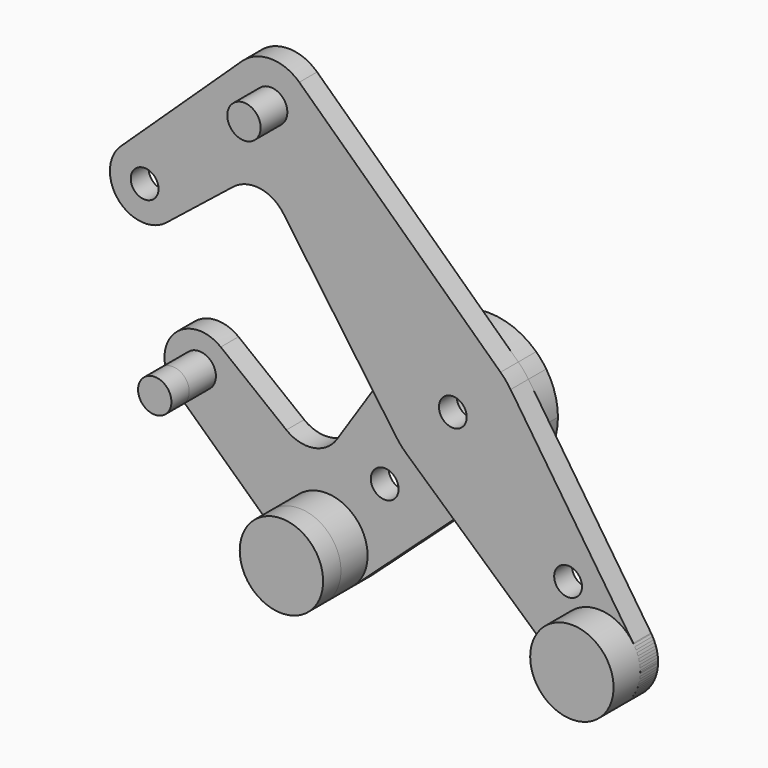
from build123d import *

# Parameters (mm, degrees)
F0_R     = 3.175
F0_R_2   = 3.96875
F2_DEPTH = 5.08
F3_DEPTH = 5.08
F4_R     = 3.81
F6_DEPTH = 12.7
F4_R_2   = 9.525
F5_R     = 3.81
F5_R_2   = 9.525


# Not quite as in the source:
# - a pattern or mirror of a feature is missing from the dataset's text; its kind, count and spacing are read off the source's solid


with BuildPart() as f2:
    # F0 (on Front) → F2 (new body)
    with BuildSketch(Plane.XZ):
        with BuildLine():
            ThreePointArc((-62.4511918078, 23.0063483758), (-67.2442419203, 30.2944442282), (-75.8348368232, 28.7807237291))
            ThreePointArc((-75.8348368232, 28.7807237291), (-76.3849752141, 17.8055319436), (-65.4422370763, 16.798571653))
            ThreePointArc((-65.4422370763, 16.798571653), (-63.237943921, 19.5609585706), (-62.4511918078, 23.0063483758))
        make_face()
        with Locations((-70.3886918078, 23.0063483758)):
            Circle(F0_R, mode=Mode.SUBTRACT)
        with BuildLine():
            ThreePointArc((-13.2524193062, 8.7400805221), (-1.834314477, 15.7686687897), (10.8922900307, 11.5487507067))
            Line((10.8922900307, 11.5487507067), (-35.0711574392, 54.8995176744))
            ThreePointArc((-35.0711574392, 54.8995176744), (-32.8608164346, 51.7436071154), (-32.0815314576, 47.9702672503))
            ThreePointArc((-32.0815314576, 47.9702672503), (-45.3798713227, 39.2245522274), (-48.1419054761, 54.8995176744))
            Line((-48.1419054761, 54.8995176744), (-75.8348368232, 28.7807237291))
            ThreePointArc((-75.8348368232, 28.7807237291), (-67.2442419203, 30.2944442282), (-62.4511918078, 23.0063483758))
            ThreePointArc((-62.4511918078, 23.0063483758), (-63.237943921, 19.5609585706), (-65.4422370763, 16.798571653))
            Line((-65.4422370763, 16.798571653), (-50.1509863937, 28.9828821829))
            ThreePointArc((-50.1509863937, 28.9828821829), (-44.0823996147, 30.6328866939), (-38.7182233604, 27.3502241323))
            Line((-38.7182233604, 27.3502241323), (-19.2147683858, -0.3005169703))
            Line((-19.2147683858, -0.3005169703), (-13.2524193062, 8.7400805221))
        make_face()
        with BuildLine():
            ThreePointArc((-32.0815314576, 47.9702672503), (-32.8608164346, 51.7436071154), (-35.0711574392, 54.8995176744))
            ThreePointArc((-35.0711574392, 54.8995176744), (-41.6065314576, 57.4952672503), (-48.1419054761, 54.8995176744))
            ThreePointArc((-48.1419054761, 54.8995176744), (-45.3798713227, 39.2245522274), (-32.0815314576, 47.9702672503))
        make_face()
        with Locations((-41.6065314576, 47.9702672503)):
            Circle(F0_R, mode=Mode.SUBTRACT)
        with BuildLine():
            ThreePointArc((15.875, 0), (15.1912005478, 4.609018433), (13.1987101208, 8.820979319))
            ThreePointArc((13.1987101208, 8.820979319), (12.1224690662, 10.2499448164), (10.8922900307, 11.5487507067))
            ThreePointArc((10.8922900307, 11.5487507067), (-1.834314477, 15.7686687897), (-13.2524193062, 8.7400805221))
            ThreePointArc((-13.2524193062, 8.7400805221), (-15.8730587934, -0.2482529814), (-12.9726166036, -9.1502373442))
            ThreePointArc((-12.9726166036, -9.1502373442), (-11.8607666217, -10.5516747555), (-10.5983019047, -11.8191210221))
            ThreePointArc((-10.5983019047, -11.8191210221), (0.0485522706, -15.8749257534), (10.6703987497, -11.7540722953))
            ThreePointArc((10.6703987497, -11.7540722953), (14.5156502636, -6.4274040191), (15.875, 0))
        make_face()
        Circle(F0_R_2, mode=Mode.SUBTRACT)
        with BuildLine():
            ThreePointArc((-12.9726166036, -9.1502373442), (-15.8730587934, -0.2482529814), (-13.2524193062, 8.7400805221))
            Line((-13.2524193062, 8.7400805221), (-19.2147683858, -0.3005169703))
            Line((-19.2147683858, -0.3005169703), (-12.9726166036, -9.1502373442))
        make_face()
        with BuildLine():
            Line((-10.5983019047, -11.8191210221), (0.0653932355, -21.3813431455))
            Line((0.0653932355, -21.3813431455), (10.6703987497, -11.7540722953))
            ThreePointArc((10.6703987497, -11.7540722953), (0.0485522706, -15.8749257534), (-10.5983019047, -11.8191210221))
        make_face()
        with BuildLine():
            ThreePointArc((26.9262440233, -45.4676864135), (27.0442454474, -31.1806737127), (41.2044512386, -33.0836262089))
            Line((41.2044512386, -33.0836262089), (13.1987101208, 8.820979319))
            ThreePointArc((13.1987101208, 8.820979319), (15.1912005478, 4.609018433), (15.875, 0))
            ThreePointArc((15.875, 0), (14.5156502636, -6.4274040191), (10.6703987497, -11.7540722953))
            Line((10.6703987497, -11.7540722953), (0.0653932355, -21.3813431455))
            Line((0.0653932355, -21.3813431455), (26.9262440233, -45.4676864135))
        make_face()
        with Locations((26.3222689506, -25.5025770961)):
            Circle(F0_R, mode=Mode.SUBTRACT)
        with BuildLine():
            ThreePointArc((26.9262440233, -45.4676864135), (37.1682864336, -47.0737686401), (42.8102251661, -38.3762138003))
            ThreePointArc((42.8102251661, -38.3762138003), (42.3999454948, -35.6108027404), (41.2044512386, -33.0836262089))
            ThreePointArc((41.2044512386, -33.0836262089), (27.0442454474, -31.1806737127), (26.9262440233, -45.4676864135))
        make_face()
        with Locations((33.2852251661, -38.3762138003)):
            Circle(F0_R, mode=Mode.SUBTRACT)
        Circle(F0_R_2)
        Circle(F0_R, mode=Mode.SUBTRACT)
    extrude(amount=F2_DEPTH)


with BuildPart() as f3:
    # F0 (on Front) → F3 (new body)
    with BuildSketch(Plane.XZ):
        with BuildLine():
            ThreePointArc((15.875, 0), (15.1912005478, 4.609018433), (13.1987101208, 8.820979319))
            ThreePointArc((13.1987101208, 8.820979319), (12.1224690662, 10.2499448164), (10.8922900307, 11.5487507067))
            ThreePointArc((10.8922900307, 11.5487507067), (-1.834314477, 15.7686687897), (-13.2524193062, 8.7400805221))
            ThreePointArc((-13.2524193062, 8.7400805221), (-15.8730587934, -0.2482529814), (-12.9726166036, -9.1502373442))
            ThreePointArc((-12.9726166036, -9.1502373442), (-11.8607666217, -10.5516747555), (-10.5983019047, -11.8191210221))
            ThreePointArc((-10.5983019047, -11.8191210221), (0.0485522706, -15.8749257534), (10.6703987497, -11.7540722953))
            ThreePointArc((10.6703987497, -11.7540722953), (14.5156502636, -6.4274040191), (15.875, 0))
        make_face()
        Circle(F0_R_2, mode=Mode.SUBTRACT)
        with BuildLine():
            Line((-10.5983019047, -11.8191210221), (0.0653932355, -21.3813431455))
            Line((0.0653932355, -21.3813431455), (10.6703987497, -11.7540722953))
            ThreePointArc((10.6703987497, -11.7540722953), (0.0485522706, -15.8749257534), (-10.5983019047, -11.8191210221))
        make_face()
        with BuildLine():
            Line((-26.647623873, -45.6315380732), (0.0653932355, -21.3813431455))
            Line((0.0653932355, -21.3813431455), (-10.5983019047, -11.8191210221))
            ThreePointArc((-10.5983019047, -11.8191210221), (-11.8607666217, -10.5516747555), (-12.9726166036, -9.1502373442))
            Line((-12.9726166036, -9.1502373442), (-19.2147683858, -0.3005169703))
            Line((-19.2147683858, -0.3005169703), (-30.5474012326, -17.4839744853))
            ThreePointArc((-30.5474012326, -17.4839744853), (-35.9047663103, -20.9493627188), (-42.0820013957, -19.3518512525))
            Line((-42.0820013957, -19.3518512525), (-57.0757936348, -7.5537803256))
            ThreePointArc((-57.0757936348, -7.5537803256), (-54.8440071189, -10.3244537385), (-54.0466841448, -13.7916973539))
            ThreePointArc((-54.0466841448, -13.7916973539), (-58.817458973, -21.070142101), (-67.394906617, -19.5992776228))
            Line((-67.394906617, -19.5992776228), (-39.5427300894, -45.5481910186))
            ThreePointArc((-39.5427300894, -45.5481910186), (-36.849933329, -29.8449609995), (-23.5248631228, -38.579094696))
            ThreePointArc((-23.5248631228, -38.579094696), (-24.3404729646, -42.4355371074), (-26.647623873, -45.6315380732))
        make_face()
        with Locations((-19.6233562292, -22.9063374758)):
            Circle(F0_R, mode=Mode.SUBTRACT)
        with BuildLine():
            ThreePointArc((-12.9726166036, -9.1502373442), (-15.8730587934, -0.2482529814), (-13.2524193062, 8.7400805221))
            Line((-13.2524193062, 8.7400805221), (-19.2147683858, -0.3005169703))
            Line((-19.2147683858, -0.3005169703), (-12.9726166036, -9.1502373442))
        make_face()
        with BuildLine():
            ThreePointArc((-57.0757936348, -7.5537803256), (-68.0121676911, -8.627656241), (-67.394906617, -19.5992776228))
            ThreePointArc((-67.394906617, -19.5992776228), (-58.817458973, -21.070142101), (-54.0466841448, -13.7916973539))
            ThreePointArc((-54.0466841448, -13.7916973539), (-54.8440071189, -10.3244537385), (-57.0757936348, -7.5537803256))
        make_face()
        with Locations((-61.9841841448, -13.7916973539)):
            Circle(F0_R, mode=Mode.SUBTRACT)
        with BuildLine():
            ThreePointArc((-39.5427300894, -45.5481910186), (-33.1114263313, -48.1038957423), (-26.647623873, -45.6315380732))
            ThreePointArc((-26.647623873, -45.6315380732), (-24.3404729646, -42.4355371074), (-23.5248631228, -38.579094696))
            ThreePointArc((-23.5248631228, -38.579094696), (-36.849933329, -29.8449609995), (-39.5427300894, -45.5481910186))
        make_face()
        with Locations((-33.0498631228, -38.579094696)):
            Circle(F0_R, mode=Mode.SUBTRACT)
    extrude(amount=-F3_DEPTH)


with BuildPart() as f6:
    # F4 (on face) → F6 (new body, through all)
    with BuildSketch(Plane(origin=(0, 0, 0), x_dir=(-1, 0, 0), z_dir=(0, 1, 0))):
        with Locations((41.6065314576, 47.9702672503)):
            Circle(F4_R)
    extrude(amount=-F6_DEPTH)


with BuildPart() as f6b:
    # F4 (on face) → F6, piece 2 (new body, through all)
    with BuildSketch(Plane(origin=(0, 0, 0), x_dir=(-1, 0, 0), z_dir=(0, 1, 0))):
        with Locations((-33.2852251661, -38.3762138003)):
            Circle(F4_R_2)
    extrude(amount=-F6_DEPTH)


with BuildPart() as f6c:
    # F5 (on face) → F6, piece 3 (new body, through all)
    with BuildSketch(Plane(origin=(0, 5.08, 0), x_dir=(-1, 0, 0), z_dir=(0, 1, 0))):
        with Locations((61.9841841448, -13.7916973539)):
            Circle(F5_R)
    extrude(amount=-F6_DEPTH)

    # F6_3_copies: F6c across plane


with BuildPart() as f6d:
    # F5 (on face) → F6, piece 4 (new body, through all)
    with BuildSketch(Plane(origin=(0, 5.08, 0), x_dir=(-1, 0, 0), z_dir=(0, 1, 0))):
        with Locations((33.0498631228, -38.579094696)):
            Circle(F5_R_2)
    extrude(amount=-F6_DEPTH)

    # F6_4_copies: F6d across plane


with BuildPart() as f6c_1:
    add(f6c.part)
    add(f6c.part.mirror(Plane(origin=(0, -3.81, 0), x_dir=(0, 0, -1), z_dir=(0, -1, 0))))


with BuildPart() as f6d_1:
    add(f6d.part)
    add(f6d.part.mirror(Plane(origin=(0, -3.81, 0), x_dir=(0, 0, -1), z_dir=(0, -1, 0))))


solid = Compound([f2.part, f3.part, f6.part, f6b.part, f6c_1.part, f6d_1.part])
